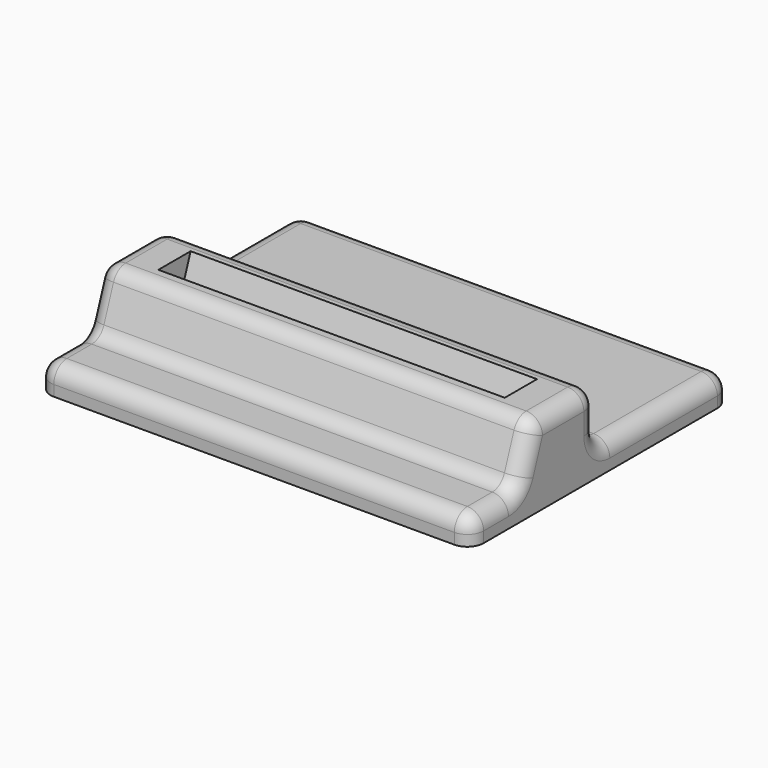
from build123d import *

# Parameters (mm, degrees)
F0_W     = 101.6
F0_H     = 76.2
F1_DEPTH = 19.05
F3_W     = 81.28
F3_H     = 8.89
F4_DEPTH = 31.75
F5_W     = 39.1665739621
F5_H     = 12.7
F6_DEPTH = 101.601
F7_F1_R  = 3.81
F7_F2_R  = 3.81


with BuildPart() as f1:
    # F0 (on Top) → F1 (new body)
    with BuildSketch(Plane.XY):
        with Locations((-4.0153246373, -5.6604754616)):
            Rectangle(F0_W, F0_H)
    extrude(amount=F1_DEPTH)

    # F3 (on face) → F4 (cut)
    with BuildSketch(Plane(origin=(0, 9.9172554964, 27.2474355394), x_dir=(1, 0, 0), z_dir=(0, 0.3420201433, 0.9396926208))):
        with Locations((-4.0153246373, -21.8419839543)):
            Rectangle(F3_W, F3_H)
    extrude(amount=-F4_DEPTH, mode=Mode.SUBTRACT)

    # F5 (on face) → F6 (cut, through all)
    with BuildSketch(Plane.YZ.offset(46.7846753627)):
        Polygon((-29.9731970935, 6.35), (-25.3507751184, 19.05), (-43.7604754616, 19.05), (-43.7604754616, 6.35), align=None)
        with Locations((12.8562375574, 12.7)):
            Rectangle(F5_W, F5_H)
    extrude(amount=-F6_DEPTH, mode=Mode.SUBTRACT)

    # F7: fillet of radius 3.81 on 19 edges, made by hand

    # F7_f1
    f7_f1_edges = [f1.edges().sort_by_distance(p)[0] for p in [
        (-4.0153246373, -29.9731970935, 6.35),
        (-4.0153246373, -6.7270494237, 6.35),
    ]]
    fillet(f7_f1_edges, radius=F7_F1_R)

    # F7_f2
    f7_f2_edges = [f1.edges().sort_by_distance(p)[0] for p in [
        (-4.0153246373, -25.3507751184, 19.05),
        (-4.0153246373, -6.7270494237, 19.05),
        (46.7846753627, -38.2007316379, 6.35),
        (-4.0153246373, -43.7604754616, 6.35),
        (-54.8153246373, -38.2007316379, 6.35),
        (-54.8153246373, 14.7612375574, 6.35),
        (-4.0153246373, 32.4395245384, 6.35),
        (46.7846753627, 14.7612375574, 6.35),
        (46.7846753627, 32.4395245384, 3.175),
        (46.7846753627, -43.7604754616, 3.175),
        (-54.8153246373, -43.7604754616, 3.175),
        (-54.8153246373, -27.2057670236, 13.953451627),
        (-54.8153246373, -6.7270494237, 14.605),
        (46.7846753627, -27.2057670236, 13.953451627),
        (46.7846753627, -16.038912271, 19.05),
        (-54.8153246373, -16.038912271, 19.05),
        (-54.8153246373, 32.4395245384, 3.175),
        (46.7846753627, -30.4556615916, 7.0390307113),
        (-54.8153246373, -5.61112626, 7.4659231637),
        (-54.8153246373, -30.4556615916, 7.0390307113),
        (46.7846753627, -5.61112626, 7.4659231637),
    ]]
    fillet(f7_f2_edges, radius=F7_F2_R)


solid = f1.part
